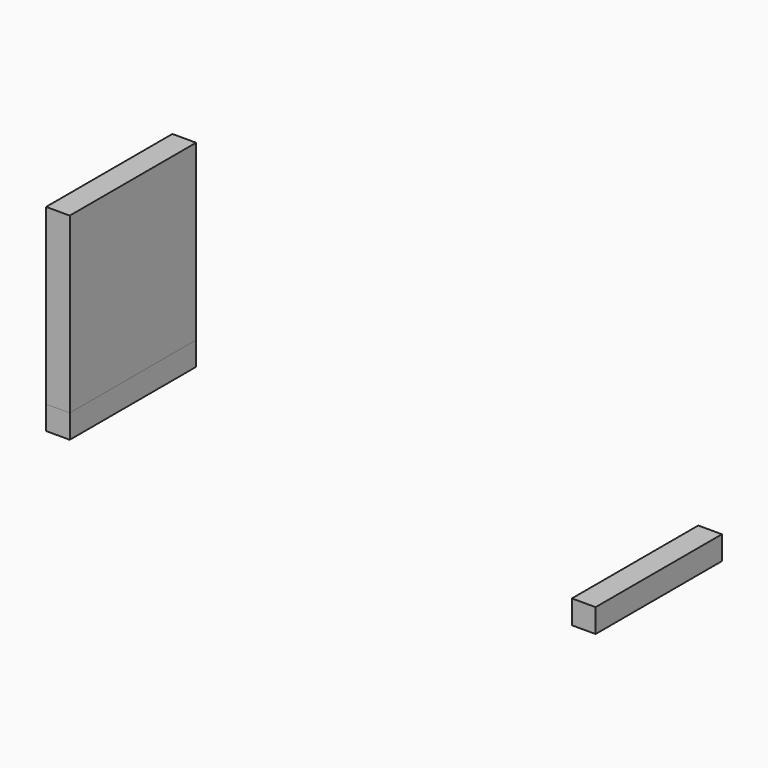
from build123d import *

# Parameters (mm, degrees)
F0_W     = 12
F0_H     = 80
F1_DEPTH = 100
F2_DEPTH = 12
F3_DEPTH = 12


# Not quite as in the source:
# - a feature names something its author has since deleted; it is built from what else it names


with BuildPart() as f1:
    # F0 (on Top) → F1 (new body)
    with BuildSketch(Plane.XY):
        with Locations((-49.4798701257, -0.5611437102)):
            Rectangle(F0_W, F0_H)
    extrude(amount=F1_DEPTH)

    # F0 (on Top) → F2 (join)
    with BuildSketch(Plane.XY):
        with Locations((-49.4798701257, -0.5611437102)):
            Rectangle(F0_W, F0_H)
    extrude(amount=F2_DEPTH)


with BuildPart() as f2:
    # F0 (on Top) → F2, piece 2 (new body)
    with BuildSketch(Plane.XY):
        with Locations((216.9306901693, -0.5611433089)):
            Rectangle(F0_W, F0_H)
    extrude(amount=F2_DEPTH)


with BuildPart() as f3:
    # F0 (on Top) → F3 (new body)
    with BuildSketch(Plane.XY):
        with Locations((-49.4798701257, -0.5611437102)):
            Rectangle(F0_W, F0_H)
    extrude(amount=F3_DEPTH)


with BuildPart() as f3b:
    # F0 (on Top) → F3, piece 2 (new body)
    with BuildSketch(Plane.XY):
        with Locations((216.9306901693, -0.5611433089)):
            Rectangle(F0_W, F0_H)
    extrude(amount=F3_DEPTH)


solid = Compound([f1.part, f2.part, f3.part, f3b.part])
